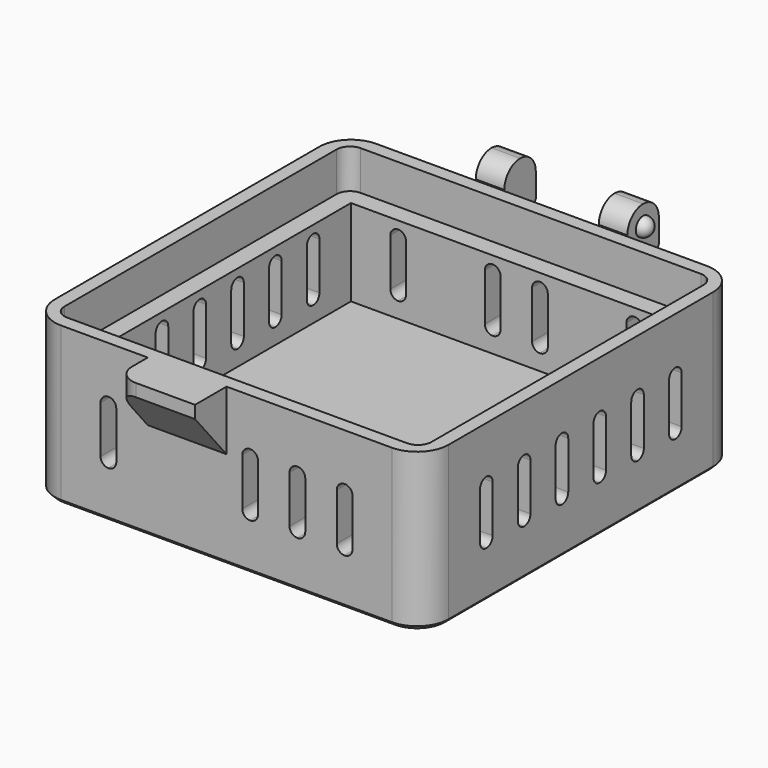
from build123d import *

# Parameters (mm, degrees)
F0_W         = 50
F0_H         = 50
F1_DEPTH     = 20
F2_T         = -4
F3_R         = 4
F5_DEPTH     = 50
F7_DEPTH     = 50.001
F8_W         = 46.6
F8_H         = 46.6
F9_DEPTH     = 5
F10_R        = 1.7
F12_DEPTH    = 3.675
F14_DEPTH    = 9.625
F15_T1_DEPTH = 31.75
F18_W        = 12
F18_H        = 10
F19_DEPTH    = 25
F20_W        = 4
F20_H        = 10
F21_DEPTH    = 4
F22_W        = 12
F22_H        = 10
F23_DEPTH    = 4
F25_DEPTH    = 10
F26_SIZE     = 0.5
F27_R        = 2.5


# Not quite as in the source:
# - a fillet or chamfer that OpenCascade refuses, or shapes differently, is made with other operations: its cross-section is extruded or revolved along the edge and cut away or added
# - a pattern or mirror of a feature is missing from the dataset's text; its kind, count and spacing are read off the source's solid


with BuildPart() as f1:
    # F0 (on Top) → F1 (new body)
    with BuildSketch(Plane.XY):
        Rectangle(F0_W, F0_H)
    extrude(amount=F1_DEPTH)

    # F2
    f2_openings = [f1.faces().sort_by_distance(p)[0] for p in [
        (0, 0, 20),
    ]]
    offset(amount=F2_T, openings=f2_openings)

    # F3
    f3_edges = [f1.edges().sort_by_distance(p)[0] for p in [
        (-25, -25, 10),
        (25, -25, 10),
        (25, 25, 10),
        (-25, 25, 10),
    ]]
    fillet(f3_edges, radius=F3_R)

    # F4 (on face) → F5 (cut)
    with BuildSketch(Plane.XZ.offset(25)):
        with BuildLine():
            ThreePointArc((-15, 6), (-14.2928932188, 6.2928932188), (-14, 7))
            Line((-14, 7), (-14, 13))
            ThreePointArc((-14, 13), (-14.2928932188, 13.7071067812), (-15, 14))
            ThreePointArc((-15, 14), (-15.7071067812, 13.7071067812), (-16, 13))
            Line((-16, 13), (-16, 7))
            ThreePointArc((-16, 7), (-15.7071067812, 6.2928932188), (-15, 6))
        make_face()
        with BuildLine():
            Line((-10, 13), (-10, 7))
            ThreePointArc((-10, 7), (-9.7071067812, 6.2928932188), (-9, 6))
            ThreePointArc((-9, 6), (-8.2928932188, 6.2928932188), (-8, 7))
            Line((-8, 7), (-8, 13))
            ThreePointArc((-8, 13), (-8.2928932188, 13.7071067812), (-9, 14))
            ThreePointArc((-9, 14), (-9.7071067812, 13.7071067812), (-10, 13))
        make_face()
        with BuildLine():
            Line((-4, 13), (-4, 7))
            ThreePointArc((-4, 7), (-3.7071067812, 6.2928932188), (-3, 6))
            ThreePointArc((-3, 6), (-2.2928932188, 6.2928932188), (-2, 7))
            Line((-2, 7), (-2, 13))
            ThreePointArc((-2, 13), (-2.2928932188, 13.7071067812), (-3, 14))
            ThreePointArc((-3, 14), (-3.7071067812, 13.7071067812), (-4, 13))
        make_face()
        with BuildLine():
            Line((2, 13), (2, 7))
            ThreePointArc((2, 7), (2.2928932188, 6.2928932188), (3, 6))
            ThreePointArc((3, 6), (3.7071067812, 6.2928932188), (4, 7))
            Line((4, 7), (4, 13))
            ThreePointArc((4, 13), (3.7071067812, 13.7071067812), (3, 14))
            ThreePointArc((3, 14), (2.2928932188, 13.7071067812), (2, 13))
        make_face()
        with BuildLine():
            Line((8, 13), (8, 7))
            ThreePointArc((8, 7), (8.2928932188, 6.2928932188), (9, 6))
            ThreePointArc((9, 6), (9.7071067812, 6.2928932188), (10, 7))
            Line((10, 7), (10, 13))
            ThreePointArc((10, 13), (9.7071067812, 13.7071067812), (9, 14))
            ThreePointArc((9, 14), (8.2928932188, 13.7071067812), (8, 13))
        make_face()
        with BuildLine():
            ThreePointArc((15, 6), (15.7071067812, 6.2928932188), (16, 7))
            Line((16, 7), (16, 13))
            ThreePointArc((16, 13), (15.7071067812, 13.7071067812), (15, 14))
            ThreePointArc((15, 14), (14.2928932188, 13.7071067812), (14, 13))
            Line((14, 13), (14, 7))
            ThreePointArc((14, 7), (14.2928932188, 6.2928932188), (15, 6))
        make_face()
    extrude(amount=-F5_DEPTH, mode=Mode.SUBTRACT)

    # F6 (on face) → F7 (cut, through all)
    with BuildSketch(Plane.YZ.offset(25)):
        with BuildLine():
            ThreePointArc((-15, 6), (-14.2928932188, 6.2928932188), (-14, 7))
            Line((-14, 7), (-14, 13))
            ThreePointArc((-14, 13), (-14.2928932188, 13.7071067812), (-15, 14))
            ThreePointArc((-15, 14), (-15.7071067812, 13.7071067812), (-16, 13))
            Line((-16, 13), (-16, 7))
            ThreePointArc((-16, 7), (-15.7071067812, 6.2928932188), (-15, 6))
        make_face()
        with BuildLine():
            Line((-10, 13), (-10, 7))
            ThreePointArc((-10, 7), (-9.7071067812, 6.2928932188), (-9, 6))
            ThreePointArc((-9, 6), (-8.2928932188, 6.2928932188), (-8, 7))
            Line((-8, 7), (-8, 13))
            ThreePointArc((-8, 13), (-8.2928932188, 13.7071067812), (-9, 14))
            ThreePointArc((-9, 14), (-9.7071067812, 13.7071067812), (-10, 13))
        make_face()
        with BuildLine():
            Line((-4, 13), (-4, 7))
            ThreePointArc((-4, 7), (-3.7071067812, 6.2928932188), (-3, 6))
            ThreePointArc((-3, 6), (-2.2928932188, 6.2928932188), (-2, 7))
            Line((-2, 7), (-2, 13))
            ThreePointArc((-2, 13), (-2.2928932188, 13.7071067812), (-3, 14))
            ThreePointArc((-3, 14), (-3.7071067812, 13.7071067812), (-4, 13))
        make_face()
        with BuildLine():
            ThreePointArc((9, 6), (9.7071067812, 6.2928932188), (10, 7))
            Line((10, 7), (10, 13))
            ThreePointArc((10, 13), (9.7071067812, 13.7071067812), (9, 14))
            ThreePointArc((9, 14), (8.2928932188, 13.7071067812), (8, 13))
            Line((8, 13), (8, 7))
            ThreePointArc((8, 7), (8.2928932188, 6.2928932188), (9, 6))
        make_face()
        with BuildLine():
            ThreePointArc((15, 6), (15.7071067812, 6.2928932188), (16, 7))
            Line((16, 7), (16, 13))
            ThreePointArc((16, 13), (15.7071067812, 13.7071067812), (15, 14))
            ThreePointArc((15, 14), (14.2928932188, 13.7071067812), (14, 13))
            Line((14, 13), (14, 7))
            ThreePointArc((14, 7), (14.2928932188, 6.2928932188), (15, 6))
        make_face()
        with BuildLine():
            ThreePointArc((3, 14), (2.2928932188, 13.7071067812), (2, 13))
            Line((2, 13), (2, 7))
            ThreePointArc((2, 7), (2.2928932188, 6.2928932188), (3, 6))
            ThreePointArc((3, 6), (3.7071067812, 6.2928932188), (4, 7))
            Line((4, 7), (4, 13))
            ThreePointArc((4, 13), (3.7071067812, 13.7071067812), (3, 14))
        make_face()
    extrude(amount=-F7_DEPTH, mode=Mode.SUBTRACT)

    # F8 (on face) → F9 (cut)
    with BuildSketch(Plane.XY.offset(20)):
        Rectangle(F8_W, F8_H)
    extrude(amount=-F9_DEPTH, mode=Mode.SUBTRACT)

    # F10
    f10_edges = [f1.edges().sort_by_distance(p)[0] for p in [
        (-23.3, 23.3, 17.5),
        (23.3, 23.3, 17.5),
        (23.3, -23.3, 17.5),
        (-23.3, -23.3, 17.5),
    ]]
    fillet(f10_edges, radius=F10_R)

    # F11 (on Right) → F12 (join, symmetric)
    with BuildSketch(Plane.YZ):
        Polygon((-21.8, 17.5), (-23.3, 18.3660254038), (-23.3, 16.6339745962), align=None)
    extrude(amount=F12_DEPTH, both=True)

    # F13 (on Right) → F14 (join, symmetric)
    with BuildSketch(Plane.YZ):
        Polygon((26.6, 19.0737604307), (25, 18.15), (25, 8.15), (31.6, 16.0155737111), (31.6, 21.5737604307), (26.6, 21.5737604307), align=None)
    extrude(amount=F14_DEPTH, both=True)

    # F15: fillet of radius 2.5 on 2 edges, made by hand

    # F15_s2 → F15_t1 (cut)
    with BuildSketch(Plane.YZ.offset(-15.875)):
        with BuildLine():
            ThreePointArc((29.1, 21.5737604307), (27.332233047, 20.8415273837), (26.6, 19.0737604307))
            Line((26.6, 19.0737604307), (26.6, 21.5737604307))
            Line((26.6, 21.5737604307), (29.1, 21.5737604307))
        make_face()
        with BuildLine():
            ThreePointArc((31.6, 19.0737604307), (30.867766953, 20.8415273837), (29.1, 21.5737604307))
            Line((29.1, 21.5737604307), (31.6, 21.5737604307))
            Line((31.6, 21.5737604307), (31.6, 19.0737604307))
        make_face()
    extrude(amount=F15_T1_DEPTH, mode=Mode.SUBTRACT)

    # F16 (on face) → F17 (revolve)
    with BuildSketch(Plane.YZ.offset(9.625)):
        with BuildLine():
            ThreePointArc((29.1, 17.9137604307), (30.26, 19.0737604307), (29.1, 20.2337604307))
            Line((29.1, 20.2337604307), (29.1, 17.9137604307))
        make_face()
    f17 = revolve(axis=Axis((9.625, 29.1, 19.0737604307), (0, 0, -1)))

    # F17_copies: F17 across plane
    add(f17.mirror(Plane(origin=(0, 0, 0), x_dir=(0, 0, -1), z_dir=(-1, 0, 0))))

    # F18 (on Top) → F19 (cut)
    with BuildSketch(Plane.XY):
        with Locations((0, 30)):
            Rectangle(F18_W, F18_H)
    extrude(amount=F19_DEPTH, mode=Mode.SUBTRACT)

    # F20 (on face) → F21 (join)
    with BuildSketch(Plane(origin=(0, 25, 0), x_dir=(-1, 0, 0), z_dir=(0, 1, 0))):
        with Locations((-9, 10)):
            Rectangle(F20_W, F20_H)
        with Locations((9, 10)):
            Rectangle(F20_W, F20_H)
    extrude(amount=-F21_DEPTH)

    # F22 (on face) → F23 (join)
    with BuildSketch(Plane.XZ.offset(25)):
        with Locations((-6, 10)):
            Rectangle(F22_W, F22_H)
    extrude(amount=-F23_DEPTH)

    # F24 (on Right) → F25 (join)
    with BuildSketch(Plane.YZ):
        Polygon((-25, 12.441232037), (-25, 20), (-30, 20), (-30, 18.4), align=None)
    extrude(amount=-F25_DEPTH)

    # F26
    f26_edges = [f1.edges().sort_by_distance(p)[0] for p in [
        (25, 0, 0),
        (0, -25, 0),
        (23.828427, -23.828427, 0),
        (23.828427, 23.828427, 0),
        (0, 25, 0),
        (-23.828427, 23.828427, 0),
        (-25, 0, 0),
        (-23.828427, -23.828427, 0),
    ]]
    chamfer(f26_edges, length=F26_SIZE)

    # F27
    f27_edges = [f1.edges().sort_by_distance(p)[0] for p in [
        (-10, -30, 19.2),
    ]]
    fillet(f27_edges, radius=F27_R)


solid = f1.part
